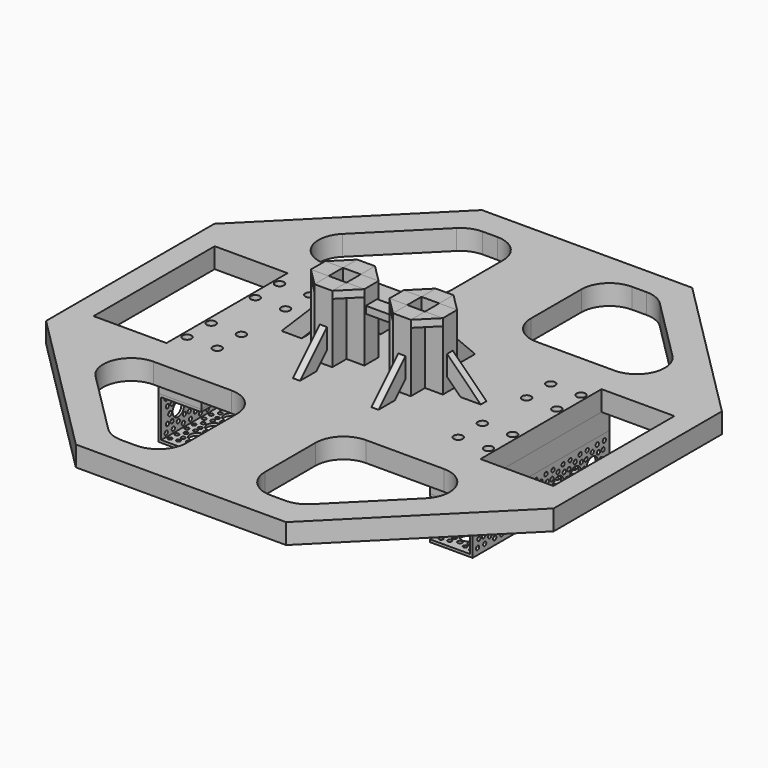
from build123d import *

# Parameters (mm, degrees)
F0_R          = 2
F1_DEPTH      = 18
F2_R          = 4
F2_R_2        = 2
F3_DEPTH      = 9
F2_W          = 15.875
F2_H          = 15.875
F4_DEPTH      = 60
F6_DEPTH      = 6.35
F8_DEPTH      = 3.175
F8_DEPTH_BACK = 3.175
F9_COUNT      = 4
F9_ANGLE      = 270
F10_COUNT     = 2
F10_ANGLE     = 90
F11_COUNT     = 2
F11_ANGLE     = 270
F13_DEPTH     = 18
F14_W         = 38.1
F14_H         = 152.4
F14_R         = 1.778
F14_R_2       = 2.032
F14_R_3       = 6.35
F15_DEPTH     = 2.286
F19_COUNT     = 3
F19_ANGLE     = 180
F12_W         = 12.7
F12_H         = 6.35
F21_DEPTH     = 22.375


# Not quite as in the source:
# - a length typed as a fraction of an inch, garbled in the dataset ("3 / 203.2 mm" for 3/8 in), is restored


with BuildPart() as f1:
    # F0 (on Top) → F1 (new body)
    with BuildSketch(Plane.XY):
        Polygon((-93.7574409294, -226.3504854653), (93.7574409294, -226.3504854653), (226.3504854653, -93.7574409294), (226.3504854653, 93.7574409294), (93.7574409294, 226.3504854653), (-93.7574409294, 226.3504854653), (-226.3504854653, 93.7574409294), (-226.3504854653, -93.7574409294), (-225.1079263947, -95), align=None)
        with BuildLine():
            ThreePointArc((-73.0467628108, -201.3504854653), (-82.6138486199, -199.447473778), (-90.7244323405, -194.0281549949))
            Line((-90.7244323405, -194.0281549949), (-147.0749178057, -137.6776695297))
            ThreePointArc((-147.0749178057, -137.6776695297), (-152.4942365888, -110.4329141909), (-129.3972482761, -95))
            Line((-129.3972482761, -95), (-60, -95))
            ThreePointArc((-60, -95), (-42.3223304703, -102.3223304703), (-35, -120))
            Line((-35, -120), (-35, -176.3504854653))
            ThreePointArc((-35, -176.3504854653), (-42.3223304703, -194.0281549949), (-60, -201.3504854653))
            Line((-60, -201.3504854653), (-73.0467628108, -201.3504854653))
        make_face(mode=Mode.SUBTRACT)
        with BuildLine():
            Line((147.0749178057, -137.6776695297), (90.7244323405, -194.0281549949))
            ThreePointArc((90.7244323405, -194.0281549949), (82.6138486199, -199.447473778), (73.0467628108, -201.3504854653))
            Line((73.0467628108, -201.3504854653), (60, -201.3504854653))
            ThreePointArc((60, -201.3504854653), (42.3223304703, -194.0281549949), (35, -176.3504854653))
            Line((35, -176.3504854653), (35, -120))
            ThreePointArc((35, -120), (42.3223304703, -102.3223304703), (60, -95))
            Line((60, -95), (129.3972482761, -95))
            ThreePointArc((129.3972482761, -95), (152.4942365888, -110.4329141909), (147.0749178057, -137.6776695297))
        make_face(mode=Mode.SUBTRACT)
        Polygon((-205, -67.5), (-205, 67.5), (-140, 67.5), (-140, 76.2), (-101.9, 76.2), (-101.9, -76.2), (-140, -76.2), (-140, -67.5), align=None, mode=Mode.SUBTRACT)
        with BuildLine():
            Line((-73.0467628108, 201.3504854653), (-60, 201.3504854653))
            ThreePointArc((-60, 201.3504854653), (-42.3223304703, 194.0281549949), (-35, 176.3504854653))
            Line((-35, 176.3504854653), (-35, 120))
            ThreePointArc((-35, 120), (-42.3223304703, 102.3223304703), (-60, 95))
            Line((-60, 95), (-129.3972482761, 95))
            ThreePointArc((-129.3972482761, 95), (-152.4942365888, 110.4329141909), (-147.0749178057, 137.6776695297))
            Line((-147.0749178057, 137.6776695297), (-90.7244323405, 194.0281549949))
            ThreePointArc((-90.7244323405, 194.0281549949), (-82.6138486199, 199.447473778), (-73.0467628108, 201.3504854653))
        make_face(mode=Mode.SUBTRACT)
        Polygon((140, 67.5), (205, 67.5), (205, -67.5), (140, -67.5), (140, -76.2), (101.9, -76.2), (101.9, 76.2), (140, 76.2), align=None, mode=Mode.SUBTRACT)
        with BuildLine():
            ThreePointArc((35, 176.3504854653), (42.3223304703, 194.0281549949), (60, 201.3504854653))
            Line((60, 201.3504854653), (73.0467628108, 201.3504854653))
            ThreePointArc((73.0467628108, 201.3504854653), (82.6138486199, 199.447473778), (90.7244323405, 194.0281549949))
            Line((90.7244323405, 194.0281549949), (147.0749178057, 137.6776695297))
            ThreePointArc((147.0749178057, 137.6776695297), (152.4942365888, 110.4329141909), (129.3972482761, 95))
            Line((129.3972482761, 95), (60, 95))
            ThreePointArc((60, 95), (42.3223304703, 102.3223304703), (35, 120))
            Line((35, 120), (35, 176.3504854653))
        make_face(mode=Mode.SUBTRACT)
        Polygon((-140, 76.2), (-140, 67.5), (-140, -67.5), (-140, -76.2), (-101.9, -76.2), (-101.9, 76.2), align=None)
        with Locations((-134.412, -51.562)):
            Circle(F0_R, mode=Mode.SUBTRACT)
        with Locations((-134.412, -24.6126)):
            Circle(F0_R, mode=Mode.SUBTRACT)
        with Locations((-107.4626, -51.562)):
            Circle(F0_R, mode=Mode.SUBTRACT)
        with Locations((-107.4626, -24.6126)):
            Circle(F0_R, mode=Mode.SUBTRACT)
        with Locations((-134.412, 24.6126)):
            Circle(F0_R, mode=Mode.SUBTRACT)
        with Locations((-134.412, 51.562)):
            Circle(F0_R, mode=Mode.SUBTRACT)
        with Locations((-107.4626, 24.6126)):
            Circle(F0_R, mode=Mode.SUBTRACT)
        with Locations((-107.4626, 51.562)):
            Circle(F0_R, mode=Mode.SUBTRACT)
        Polygon((140, -67.5), (140, 67.5), (140, 76.2), (101.9, 76.2), (101.9, -76.2), (140, -76.2), align=None)
        with Locations((107.4626, -51.562)):
            Circle(F0_R, mode=Mode.SUBTRACT)
        with Locations((107.4626, -24.6126)):
            Circle(F0_R, mode=Mode.SUBTRACT)
        with Locations((134.412, -51.562)):
            Circle(F0_R, mode=Mode.SUBTRACT)
        with Locations((134.412, -24.6126)):
            Circle(F0_R, mode=Mode.SUBTRACT)
        with Locations((107.4626, 24.6126)):
            Circle(F0_R, mode=Mode.SUBTRACT)
        with Locations((107.4626, 51.562)):
            Circle(F0_R, mode=Mode.SUBTRACT)
        with Locations((134.412, 24.6126)):
            Circle(F0_R, mode=Mode.SUBTRACT)
        with Locations((134.412, 51.562)):
            Circle(F0_R, mode=Mode.SUBTRACT)
    extrude(amount=F1_DEPTH)

    # F2 (on face) → F3 (cut)
    with BuildSketch(Plane.XY.offset(18)):
        with Locations((-134.412, 51.562)):
            Circle(F2_R)
        with Locations((-134.412, 51.562)):
            Circle(F2_R_2, mode=Mode.SUBTRACT)
        with Locations((-107.4626, 51.562)):
            Circle(F2_R)
        with Locations((-107.4626, 51.562)):
            Circle(F2_R_2, mode=Mode.SUBTRACT)
        with Locations((-134.412, 24.6126)):
            Circle(F2_R)
        with Locations((-134.412, 24.6126)):
            Circle(F2_R_2, mode=Mode.SUBTRACT)
        with Locations((-107.4626, 24.6126)):
            Circle(F2_R)
        with Locations((-107.4626, 24.6126)):
            Circle(F2_R_2, mode=Mode.SUBTRACT)
        with Locations((-134.412, -24.6126)):
            Circle(F2_R)
        with Locations((-134.412, -24.6126)):
            Circle(F2_R_2, mode=Mode.SUBTRACT)
        with Locations((-107.4626, -24.6126)):
            Circle(F2_R)
        with Locations((-107.4626, -24.6126)):
            Circle(F2_R_2, mode=Mode.SUBTRACT)
        with Locations((-134.412, -51.562)):
            Circle(F2_R)
        with Locations((-134.412, -51.562)):
            Circle(F2_R_2, mode=Mode.SUBTRACT)
        with Locations((-107.4626, -51.562)):
            Circle(F2_R)
        with Locations((-107.4626, -51.562)):
            Circle(F2_R_2, mode=Mode.SUBTRACT)
        with Locations((107.4626, 51.562)):
            Circle(F2_R)
        with Locations((107.4626, 51.562)):
            Circle(F2_R_2, mode=Mode.SUBTRACT)
        with Locations((134.412, 51.562)):
            Circle(F2_R)
        with Locations((134.412, 51.562)):
            Circle(F2_R_2, mode=Mode.SUBTRACT)
        with Locations((107.4626, 24.6126)):
            Circle(F2_R)
        with Locations((107.4626, 24.6126)):
            Circle(F2_R_2, mode=Mode.SUBTRACT)
        with Locations((134.412, 24.6126)):
            Circle(F2_R)
        with Locations((134.412, 24.6126)):
            Circle(F2_R_2, mode=Mode.SUBTRACT)
        with Locations((107.4626, -24.6126)):
            Circle(F2_R)
        with Locations((107.4626, -24.6126)):
            Circle(F2_R_2, mode=Mode.SUBTRACT)
        with Locations((134.412, -24.6126)):
            Circle(F2_R)
        with Locations((134.412, -24.6126)):
            Circle(F2_R_2, mode=Mode.SUBTRACT)
        with Locations((107.4626, -51.562)):
            Circle(F2_R)
        with Locations((107.4626, -51.562)):
            Circle(F2_R_2, mode=Mode.SUBTRACT)
        with Locations((134.412, -51.562)):
            Circle(F2_R)
        with Locations((134.412, -51.562)):
            Circle(F2_R_2, mode=Mode.SUBTRACT)
    extrude(amount=-F3_DEPTH, mode=Mode.SUBTRACT)


with BuildPart() as f4:
    # F2 (on face) → F4 (new body)
    with BuildSketch(Plane.XY.offset(18)):
        with Locations((-50.875, 0)):
            Rectangle(F2_W, F2_H)
    extrude(amount=F4_DEPTH)


with BuildPart() as f6:
    # F5 (on face) → F6 (new body)
    with BuildSketch(Plane.XY.offset(78)):
        Polygon((-42.9375, -23.8125), (-42.9375, -7.9375), (-58.8125, -7.9375), align=None)
    extrude(amount=-F6_DEPTH)


with BuildPart() as f8:
    # F7 (on Front) → F8 (new body, two sides)
    with BuildSketch(Plane.XZ) as f8_sk:
        Polygon((-70.8519877579, 18), (-58.8125, 30.0394877579), (-58.8125, 48), (-88.8125, 18), align=None)
    extrude(amount=F8_DEPTH)
    extrude(f8_sk.sketch, amount=-F8_DEPTH_BACK)


with BuildPart() as f9_1:
    # F9: instance of F4
    add(f4.part.rotate(Axis((-35, 0, 45.1932922006), (0, 0, 1)), 1 * F9_ANGLE / (F9_COUNT - 1)))


with BuildPart() as f9_2:
    # F9: instance of F4
    add(f4.part.rotate(Axis((-35, 0, 45.1932922006), (0, 0, 1)), 2 * F9_ANGLE / (F9_COUNT - 1)))


with BuildPart() as f9_3:
    # F9: instance of F4
    add(f4.part.rotate(Axis((-35, 0, 45.1932922006), (0, 0, 1)), 3 * F9_ANGLE / (F9_COUNT - 1)))


with BuildPart() as f9_4:
    # F9: instance of F6
    add(f6.part.rotate(Axis((-35, 0, 45.1932922006), (0, 0, 1)), 1 * F9_ANGLE / (F9_COUNT - 1)))


with BuildPart() as f9_5:
    # F9: instance of F6
    add(f6.part.rotate(Axis((-35, 0, 45.1932922006), (0, 0, 1)), 2 * F9_ANGLE / (F9_COUNT - 1)))


with BuildPart() as f9_6:
    # F9: instance of F6
    add(f6.part.rotate(Axis((-35, 0, 45.1932922006), (0, 0, 1)), 3 * F9_ANGLE / (F9_COUNT - 1)))


with BuildPart() as f10_1:
    # F10: instance of F8
    add(f8.part.rotate(Axis((-35, 0, 45.1932922006), (0, 0, 1)), 1 * F10_ANGLE / (F10_COUNT - 1)))


with BuildPart() as f11_1:
    # F11: instance of F8
    add(f8.part.rotate(Axis((-35, 0, 45.1932922006), (0, 0, 1)), 1 * F11_ANGLE / (F11_COUNT - 1)))


with BuildPart() as f13:
    # F0 (on Top) → F13 (new body)
    with BuildSketch(Plane.XY):
        Polygon((-140, 76.2), (-140, 67.5), (-140, -67.5), (-140, -76.2), (-101.9, -76.2), (-101.9, 76.2), align=None)
        with Locations((-134.412, -51.562)):
            Circle(F0_R, mode=Mode.SUBTRACT)
        with Locations((-134.412, -24.6126)):
            Circle(F0_R, mode=Mode.SUBTRACT)
        with Locations((-107.4626, -51.562)):
            Circle(F0_R, mode=Mode.SUBTRACT)
        with Locations((-107.4626, -24.6126)):
            Circle(F0_R, mode=Mode.SUBTRACT)
        with Locations((-134.412, 24.6126)):
            Circle(F0_R, mode=Mode.SUBTRACT)
        with Locations((-134.412, 51.562)):
            Circle(F0_R, mode=Mode.SUBTRACT)
        with Locations((-107.4626, 24.6126)):
            Circle(F0_R, mode=Mode.SUBTRACT)
        with Locations((-107.4626, 51.562)):
            Circle(F0_R, mode=Mode.SUBTRACT)
    extrude(amount=-F13_DEPTH)


with BuildPart() as f15:
    # F14 (on face) → F15 (new body)
    with BuildSketch(Plane(origin=(0, 0, -18), x_dir=(1, 0, 0), z_dir=(0, 0, -1))):
        with Locations((-120.95, 0)):
            Rectangle(F14_W, F14_H)
        with Locations((-134.4203841816, -70.6203841816)):
            Circle(F14_R, mode=Mode.SUBTRACT)
        with Locations((-134.4203841816, -62.7253)):
            Circle(F14_R, mode=Mode.SUBTRACT)
        with Locations((-134.4203841816, -51.5703841816)):
            Circle(F14_R, mode=Mode.SUBTRACT)
        with Locations((-130.729, -57.15)):
            Circle(F14_R, mode=Mode.SUBTRACT)
        with Locations((-134.4203841816, -43.6753)):
            Circle(F14_R, mode=Mode.SUBTRACT)
        with Locations((-127.8588, -69.2912)):
            Circle(F14_R, mode=Mode.SUBTRACT)
        with Locations((-127.8647972132, -64.0647972132)):
            Circle(F14_R, mode=Mode.SUBTRACT)
        with Locations((-127.8588, -50.2412)):
            Circle(F14_R, mode=Mode.SUBTRACT)
        with Locations((-127.8647972132, -45.0147972132)):
            Circle(F14_R, mode=Mode.SUBTRACT)
        with Locations((-134.4203841816, -32.5203841816)):
            Circle(F14_R, mode=Mode.SUBTRACT)
        with Locations((-130.729, -38.1)):
            Circle(F14_R, mode=Mode.SUBTRACT)
        with Locations((-134.4203841816, -24.6253)):
            Circle(F14_R, mode=Mode.SUBTRACT)
        with Locations((-134.4203841816, -13.4703841816)):
            Circle(F14_R, mode=Mode.SUBTRACT)
        with Locations((-130.729, -19.05)):
            Circle(F14_R, mode=Mode.SUBTRACT)
        with Locations((-134.4203841816, -5.5753)):
            Circle(F14_R, mode=Mode.SUBTRACT)
        with Locations((-127.8588, -31.1912)):
            Circle(F14_R, mode=Mode.SUBTRACT)
        with Locations((-127.8647972132, -25.9647972132)):
            Circle(F14_R, mode=Mode.SUBTRACT)
        with Locations((-127.8588, -12.1412)):
            Circle(F14_R, mode=Mode.SUBTRACT)
        with Locations((-127.8647972132, -6.9147972132)):
            Circle(F14_R, mode=Mode.SUBTRACT)
        with Locations((-120.95, -66.929)):
            Circle(F14_R_2, mode=Mode.SUBTRACT)
        with Locations((-114.0412, -69.2912)):
            Circle(F14_R, mode=Mode.SUBTRACT)
        with Locations((-114.0352027868, -64.0647972132)):
            Circle(F14_R, mode=Mode.SUBTRACT)
        with Locations((-120.95, -57.15)):
            Circle(F14_R_3, mode=Mode.SUBTRACT)
        with Locations((-120.95, -47.879)):
            Circle(F14_R_2, mode=Mode.SUBTRACT)
        with Locations((-114.0412, -50.2412)):
            Circle(F14_R, mode=Mode.SUBTRACT)
        with Locations((-114.0352027868, -45.0147972132)):
            Circle(F14_R, mode=Mode.SUBTRACT)
        with Locations((-107.4796158184, -70.6203841816)):
            Circle(F14_R, mode=Mode.SUBTRACT)
        with Locations((-107.4796158184, -62.7253)):
            Circle(F14_R, mode=Mode.SUBTRACT)
        with Locations((-111.171, -57.15)):
            Circle(F14_R, mode=Mode.SUBTRACT)
        with Locations((-107.4796158184, -51.5703841816)):
            Circle(F14_R, mode=Mode.SUBTRACT)
        with Locations((-107.4796158184, -43.6753)):
            Circle(F14_R, mode=Mode.SUBTRACT)
        with Locations((-120.95, -38.1)):
            Circle(F14_R_3, mode=Mode.SUBTRACT)
        with Locations((-120.95, -28.829)):
            Circle(F14_R_2, mode=Mode.SUBTRACT)
        with Locations((-114.0412, -31.1912)):
            Circle(F14_R, mode=Mode.SUBTRACT)
        with Locations((-114.0352027868, -25.9647972132)):
            Circle(F14_R, mode=Mode.SUBTRACT)
        with Locations((-120.95, -19.05)):
            Circle(F14_R_3, mode=Mode.SUBTRACT)
        with Locations((-120.95, -9.779)):
            Circle(F14_R_2, mode=Mode.SUBTRACT)
        with Locations((-114.0412, -12.1412)):
            Circle(F14_R, mode=Mode.SUBTRACT)
        with Locations((-114.0352027868, -6.9147972132)):
            Circle(F14_R, mode=Mode.SUBTRACT)
        with Locations((-111.171, -38.1)):
            Circle(F14_R, mode=Mode.SUBTRACT)
        with Locations((-107.4796158184, -32.5203841816)):
            Circle(F14_R, mode=Mode.SUBTRACT)
        with Locations((-107.4796158184, -24.6253)):
            Circle(F14_R, mode=Mode.SUBTRACT)
        with Locations((-111.171, -19.05)):
            Circle(F14_R, mode=Mode.SUBTRACT)
        with Locations((-107.4796158184, -13.4703841816)):
            Circle(F14_R, mode=Mode.SUBTRACT)
        with Locations((-107.4796158184, -5.5753)):
            Circle(F14_R, mode=Mode.SUBTRACT)
        with Locations((-134.4203841816, 5.5796158184)):
            Circle(F14_R, mode=Mode.SUBTRACT)
        with Locations((-130.729, 0)):
            Circle(F14_R, mode=Mode.SUBTRACT)
        with Locations((-134.4203841816, 13.4747)):
            Circle(F14_R, mode=Mode.SUBTRACT)
        with Locations((-134.4203841816, 24.6296158184)):
            Circle(F14_R, mode=Mode.SUBTRACT)
        with Locations((-130.729, 19.05)):
            Circle(F14_R, mode=Mode.SUBTRACT)
        with Locations((-134.4203841816, 32.5247)):
            Circle(F14_R, mode=Mode.SUBTRACT)
        with Locations((-127.8588, 6.9088)):
            Circle(F14_R, mode=Mode.SUBTRACT)
        with Locations((-127.8647972132, 12.1352027868)):
            Circle(F14_R, mode=Mode.SUBTRACT)
        with Locations((-127.8588, 25.9588)):
            Circle(F14_R, mode=Mode.SUBTRACT)
        with Locations((-127.8647972132, 31.1852027868)):
            Circle(F14_R, mode=Mode.SUBTRACT)
        with Locations((-134.4203841816, 43.6796158184)):
            Circle(F14_R, mode=Mode.SUBTRACT)
        with Locations((-130.729, 38.1)):
            Circle(F14_R, mode=Mode.SUBTRACT)
        with Locations((-134.4203841816, 51.5747)):
            Circle(F14_R, mode=Mode.SUBTRACT)
        with Locations((-134.4203841816, 62.7296158184)):
            Circle(F14_R, mode=Mode.SUBTRACT)
        with Locations((-130.729, 57.15)):
            Circle(F14_R, mode=Mode.SUBTRACT)
        with Locations((-134.4203841816, 70.6247)):
            Circle(F14_R, mode=Mode.SUBTRACT)
        with Locations((-127.8588, 45.0088)):
            Circle(F14_R, mode=Mode.SUBTRACT)
        with Locations((-127.8647972132, 50.2352027868)):
            Circle(F14_R, mode=Mode.SUBTRACT)
        with Locations((-127.8588, 64.0588)):
            Circle(F14_R, mode=Mode.SUBTRACT)
        with Locations((-127.8647972132, 69.2852027868)):
            Circle(F14_R, mode=Mode.SUBTRACT)
        with Locations((-120.95, 0)):
            Circle(F14_R_3, mode=Mode.SUBTRACT)
        with Locations((-120.95, 9.271)):
            Circle(F14_R_2, mode=Mode.SUBTRACT)
        with Locations((-114.0412, 6.9088)):
            Circle(F14_R, mode=Mode.SUBTRACT)
        with Locations((-114.0352027868, 12.1352027868)):
            Circle(F14_R, mode=Mode.SUBTRACT)
        with Locations((-120.95, 19.05)):
            Circle(F14_R_3, mode=Mode.SUBTRACT)
        with Locations((-120.95, 28.321)):
            Circle(F14_R_2, mode=Mode.SUBTRACT)
        with Locations((-114.0412, 25.9588)):
            Circle(F14_R, mode=Mode.SUBTRACT)
        with Locations((-114.0352027868, 31.1852027868)):
            Circle(F14_R, mode=Mode.SUBTRACT)
        with Locations((-111.171, 0)):
            Circle(F14_R, mode=Mode.SUBTRACT)
        with Locations((-107.4796158184, 5.5796158184)):
            Circle(F14_R, mode=Mode.SUBTRACT)
        with Locations((-107.4796158184, 13.4747)):
            Circle(F14_R, mode=Mode.SUBTRACT)
        with Locations((-111.171, 19.05)):
            Circle(F14_R, mode=Mode.SUBTRACT)
        with Locations((-107.4796158184, 24.6296158184)):
            Circle(F14_R, mode=Mode.SUBTRACT)
        with Locations((-107.4796158184, 32.5247)):
            Circle(F14_R, mode=Mode.SUBTRACT)
        with Locations((-120.95, 38.1)):
            Circle(F14_R_3, mode=Mode.SUBTRACT)
        with Locations((-120.95, 47.371)):
            Circle(F14_R_2, mode=Mode.SUBTRACT)
        with Locations((-114.0412, 45.0088)):
            Circle(F14_R, mode=Mode.SUBTRACT)
        with Locations((-114.0352027868, 50.2352027868)):
            Circle(F14_R, mode=Mode.SUBTRACT)
        with Locations((-120.95, 57.15)):
            Circle(F14_R_3, mode=Mode.SUBTRACT)
        with Locations((-120.95, 66.421)):
            Circle(F14_R_2, mode=Mode.SUBTRACT)
        with Locations((-114.0412, 64.0588)):
            Circle(F14_R, mode=Mode.SUBTRACT)
        with Locations((-114.0352027868, 69.2852027868)):
            Circle(F14_R, mode=Mode.SUBTRACT)
        with Locations((-111.171, 38.1)):
            Circle(F14_R, mode=Mode.SUBTRACT)
        with Locations((-107.4796158184, 43.6796158184)):
            Circle(F14_R, mode=Mode.SUBTRACT)
        with Locations((-107.4796158184, 51.5747)):
            Circle(F14_R, mode=Mode.SUBTRACT)
        with Locations((-111.171, 57.15)):
            Circle(F14_R, mode=Mode.SUBTRACT)
        with Locations((-107.4796158184, 62.7296158184)):
            Circle(F14_R, mode=Mode.SUBTRACT)
        with Locations((-107.4796158184, 70.6247)):
            Circle(F14_R, mode=Mode.SUBTRACT)
    extrude(amount=F15_DEPTH)

    # F19: F15 ×3 about axis
    f19_axis = Axis((-120.95, 0, -37.05), (0, -1, 0))


with BuildPart() as f15_1:
    add(f15.part)
    for i in range(1, F19_COUNT):
        add(f15.part.rotate(f19_axis, i * F19_ANGLE / (F19_COUNT - 1)))


with BuildPart() as f20_1:
    # F20: instance of F4
    add(f4.part.mirror(Plane.YZ))


with BuildPart() as f20_2:
    # F20: instance of F6
    add(f6.part.mirror(Plane.YZ))


with BuildPart() as f20_3:
    # F20: instance of F8
    add(f8.part.mirror(Plane.YZ))


with BuildPart() as f20_4:
    # F20: instance of F9_1
    add(f9_1.part.mirror(Plane.YZ))


with BuildPart() as f20_5:
    # F20: instance of F9_4
    add(f9_4.part.mirror(Plane.YZ))


with BuildPart() as f20_6:
    # F20: instance of F9_2
    add(f9_2.part.mirror(Plane.YZ))


with BuildPart() as f20_7:
    # F20: instance of F9_5
    add(f9_5.part.mirror(Plane.YZ))


with BuildPart() as f20_8:
    # F20: instance of F9_3
    add(f9_3.part.mirror(Plane.YZ))


with BuildPart() as f20_9:
    # F20: instance of F9_6
    add(f9_6.part.mirror(Plane.YZ))


with BuildPart() as f20_10:
    # F20: instance of F10_1
    add(f10_1.part.mirror(Plane.YZ))


with BuildPart() as f20_11:
    # F20: instance of F11_1
    add(f11_1.part.mirror(Plane.YZ))


with BuildPart() as f20_12:
    # F20: instance of F13
    add(f13.part.mirror(Plane.YZ))


with BuildPart() as f20_13:
    # F20: instance of F15
    add(f15_1.part.mirror(Plane.YZ))


with BuildPart() as f21:
    # F12 (on face) → F21 (new body, through all)
    with BuildSketch(Plane.YZ.offset(-11.1875)):
        with Locations((0, 61.175)):
            Rectangle(F12_W, F12_H)
    extrude(amount=F21_DEPTH)


solid = Compound([f1.part, f4.part, f6.part, f8.part, f9_1.part, f9_2.part, f9_3.part, f9_4.part, f9_5.part, f9_6.part, f10_1.part, f11_1.part, f13.part, f15_1.part, f20_1.part, f20_2.part, f20_3.part, f20_4.part, f20_5.part, f20_6.part, f20_7.part, f20_8.part, f20_9.part, f20_10.part, f20_11.part, f20_12.part, f20_13.part, f21.part])
